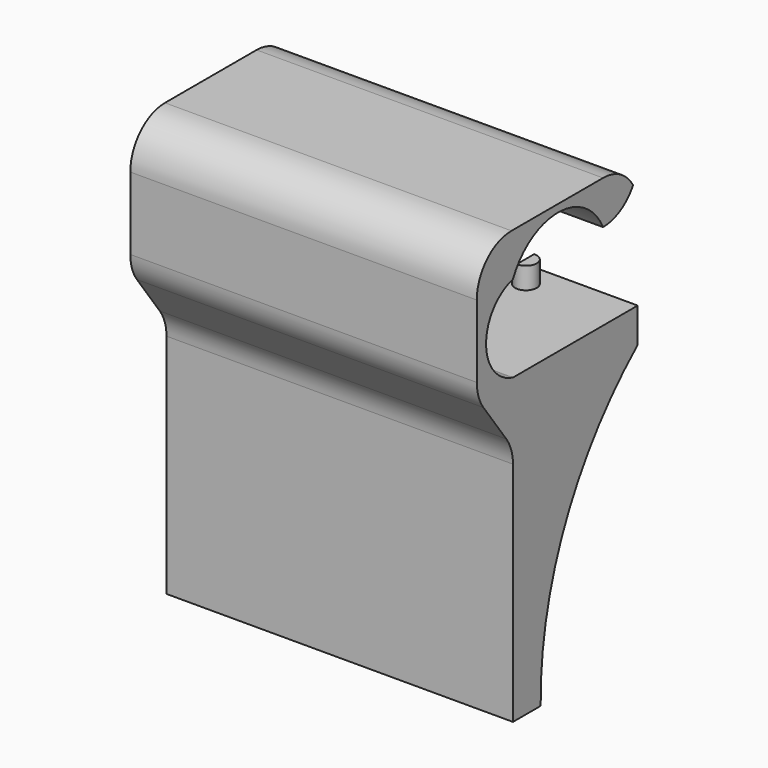
from build123d import *

# Parameters (mm, degrees)
F0_R         = 1.25
F1_DEPTH     = 2.5
F2_W         = 40
F2_H         = 18
F3_DEPTH     = 35
F5_DEPTH     = 40.001
F7_DEPTH     = 40
F9_DEPTH     = 10
F10_T1_DEPTH = 40
F10_T3_DEPTH = 65
F10_T5_DEPTH = 48.1285235511


# Not quite as in the source:
# - a fillet or chamfer that OpenCascade refuses, or shapes differently, is made with other operations: its cross-section is extruded or revolved along the edge and cut away or added


with BuildPart() as f1:
    # F0 (on Top) → F1 (new body)
    with BuildSketch(Plane.XY):
        with Locations((-9.5, 0)):
            Circle(F0_R)
    extrude(amount=F1_DEPTH)



with BuildPart() as f1b:
    # F0 (on Top) → F1, piece 2 (new body)
    with BuildSketch(Plane.XY):
        with Locations((9.5, 0)):
            Circle(F0_R)
    extrude(amount=F1_DEPTH)


with BuildPart() as f1_1:
    add(f1.part)

    add(f1b.part)  # F3 merges F1b
    # F2 (on Top) → F3 (join)
    with BuildSketch(Plane.XY):
        with Locations((0, -6)):
            Rectangle(F2_W, F2_H)
    extrude(amount=-F3_DEPTH)

    # F4 (on face) → F5 (cut, through all)
    with BuildSketch(Plane(origin=(-20, 0, 0), x_dir=(0, -1, 0), z_dir=(-1, 0, 0))):
        with BuildLine():
            Line((-3, -35), (11, -35))
            ThreePointArc((11, -35), (7.459306232, -17.9377326694), (-3, -4))
            Line((-3, -4), (-3, -35))
        make_face()
    extrude(amount=-F5_DEPTH, mode=Mode.SUBTRACT)

    # F6 (on face) → F7 (join)
    with BuildSketch(Plane(origin=(-20, 0, 0), x_dir=(0, -1, 0), z_dir=(-1, 0, 0))):
        with BuildLine():
            Line((-3, 10), (2, 10))
            ThreePointArc((2, 10), (8.5, 14.1331594945), (15, 10))
            ThreePointArc((15, 10), (18.881651405, 5), (15, 0))
            Line((15, 0), (15, -7.1779969148))
            Line((15, -7.1779969148), (20.2195104212, 0))
            Line((20.2195104212, 0), (20.2195104212, 15))
            Line((20.2195104212, 15), (-3, 15))
            Line((-3, 15), (-3, 10))
        make_face()
    extrude(amount=-F7_DEPTH)

    # F8 (on face) → F9 (cut)
    with BuildSketch(Plane(origin=(0, 3, 0), x_dir=(-1, 0, 0), z_dir=(0, 1, 0))):
        Polygon((9.1120566488, 3.2700138061), (11, 0), (11, 3.2700138061), align=None)
        Polygon((-9.8879433512, 3.2700138061), (-8, 0), (-8, 3.2700138061), align=None)
    extrude(amount=-F9_DEPTH, mode=Mode.SUBTRACT)

    # F10: fillet of radius 5 on 5 edges, made by hand

    # F10_s2 → F10_t1 (join)
    with BuildSketch(Plane.YZ.offset(-20)):
        with BuildLine():
            ThreePointArc((-15, -8.803701625), (-15.245026694, -7.257665125), (-15.9560915438, -5.8631567099))
            Line((-15.9560915438, -5.8631567099), (-15, -7.1779969148))
            Line((-15, -7.1779969148), (-15, -8.803701625))
        make_face()
    extrude(amount=F10_T1_DEPTH)

    # F10_s4 → F10_t3 (cut)
    with BuildSketch(Plane.YZ.offset(-32.5)):
        with BuildLine():
            ThreePointArc((-20.2195104212, 10), (-18.7550443271, 13.5355339059), (-15.2195104212, 15))
            Line((-15.2195104212, 15), (-20.2195104212, 15))
            Line((-20.2195104212, 15), (-20.2195104212, 10))
        make_face()
        with BuildLine():
            ThreePointArc((-2, 15), (1.5355339059, 13.5355339059), (3, 10))
            Line((3, 10), (3, 15))
            Line((3, 15), (-2, 15))
        make_face()
        with BuildLine():
            ThreePointArc((3, 15), (1.5355339059, 11.4644660941), (-2, 10))
            Line((-2, 10), (3, 10))
            Line((3, 10), (3, 15))
        make_face()
    extrude(amount=F10_T3_DEPTH, mode=Mode.SUBTRACT)

    # F10_s6 → F10_t5 (cut)
    with BuildSketch(Plane.YZ.offset(-24.0642617755)):
        with BuildLine():
            ThreePointArc((-19.2634188773, -1.314840205), (-19.9744837271, 0.0796682101), (-20.2195104212, 1.6257047102))
            Line((-20.2195104212, 1.6257047102), (-20.2195104212, 0))
            Line((-20.2195104212, 0), (-19.2634188773, -1.314840205))
        make_face()
    extrude(amount=F10_T5_DEPTH, mode=Mode.SUBTRACT)


solid = f1_1.part
